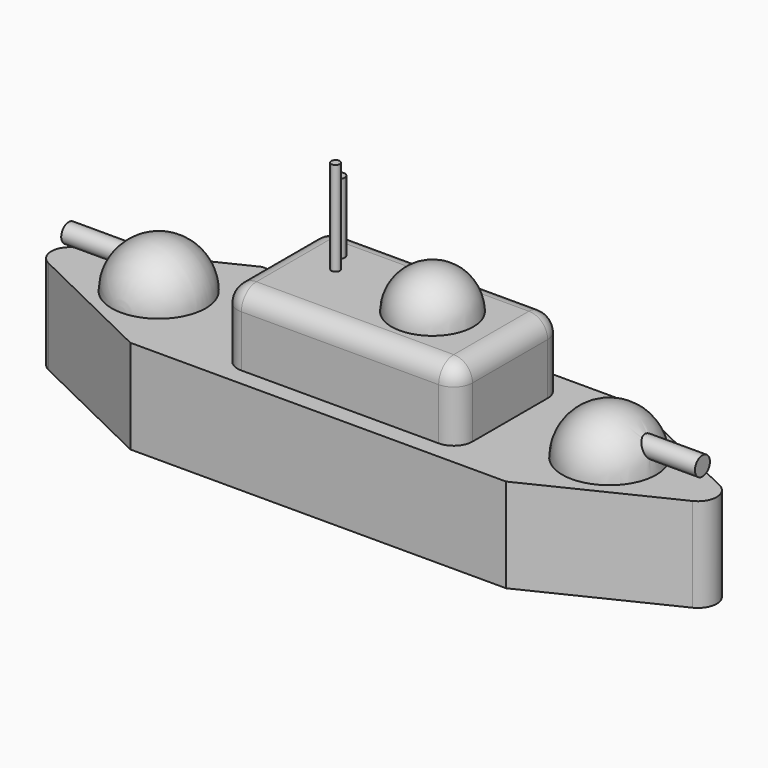
from build123d import *

# Parameters (mm, degrees)
F1_DEPTH  = 25.4
F2_W      = 63.5
F2_H      = 35.56
F3_DEPTH  = 19.05
F9_R      = 2.54
F10_DEPTH = 19.05
F12_R     = 2.54
F13_DEPTH = 19.05
F14_R     = 5.08
F15_R     = 5.08
F16_R     = 1.5271638032
F17_DEPTH = 19.05
F18_R     = 1.1438569205
F19_DEPTH = 25.4


# Not quite as in the source:
# - the program builds the solid bodies; features that only make, move or delete a surface that nothing else refers to are left out


with BuildPart() as f1:
    # F0 (on Top) → F1 (new body)
    with BuildSketch(Plane.XY):
        Polygon((-109.4730429574, -7.8658423934), (-63.7924405375, -30.0902110584), (37.8075594625, -30.0902110584), (83.4881618824, -7.8658423934), (37.8075594625, 14.3585262716), (-63.7924405375, 14.3585262716), align=None)
    extrude(amount=F1_DEPTH)

    # F2 (on face) → F3 (join)
    with BuildSketch(Plane.XY.offset(25.4)):
        with Locations((-10.9020974487, -7.5584737481)):
            Rectangle(F2_W, F2_H)
    extrude(amount=F3_DEPTH)

    # F5 (on face) → F6 (revolve)
    with BuildSketch(Plane.XY.offset(25.4)):
        with BuildLine():
            Line((-73.9079761496, 4.8341565959), (-73.9079761496, -20.5658413827))
            ThreePointArc((-73.9079761496, -20.5658413827), (-61.2130429574, -7.8658423934), (-73.9079761496, 4.8341565959))
        make_face()
    revolve(axis=Axis((-73.9079761496, -7.8658423934, 25.4), (0, 1, 0)))

    # F4 (on face) → F7 (revolve)
    with BuildSketch(Plane.XY.offset(25.4)):
        with BuildLine():
            Line((47.92816229, -7.8712259838), (47.92816229, 4.8287740162))
            ThreePointArc((47.92816229, 4.8287740162), (35.22816229, -7.8712259838), (47.92816229, -20.5712259838))
            Line((47.92816229, -20.5712259838), (47.92816229, -7.8712259838))
        make_face()
    revolve(axis=Axis((47.92816229, -7.8712259838, 25.4), (0, 1, 0)))

    # F9 (on offset) → F10 (join)
    with BuildSketch(Plane.YZ.offset(53.848)):
        with Locations((-7.6085058972, 31.3998050988)):
            Circle(F9_R)
    extrude(amount=F10_DEPTH)

    # F12 (on offset) → F13 (join)
    with BuildSketch(Plane.YZ.offset(-79.248)):
        with Locations((-7.7845989726, 31.3248895109)):
            Circle(F12_R)
    extrude(amount=-F13_DEPTH)

    # F14
    f14_edges = [f1.edges().sort_by_distance(p)[0] for p in [
        (-42.652097, -7.558474, 44.45),
        (-10.902097, -25.338474, 44.45),
        (-10.902097, 10.221526, 44.45),
        (20.847903, -7.558474, 44.45),
        (-42.652097, -25.338474, 34.925),
        (20.847903, -25.338474, 34.925),
        (20.847903, 10.221526, 34.925),
        (-42.652097, 10.221526, 34.925),
    ]]
    fillet(f14_edges, radius=F14_R)

    # F15
    f15_edges = [f1.edges().sort_by_distance(p)[0] for p in [
        (-109.473043, -7.865842, 12.7),
        (83.488162, -7.865842, 12.7),
    ]]
    fillet(f15_edges, radius=F15_R)

    # F16 (on face) → F17 (join)
    with BuildSketch(Plane.XY.offset(44.45)):
        with Locations((-31.4132720232, 0)):
            Circle(F16_R)
    extrude(amount=F17_DEPTH)

    # F18 (on face) → F19 (join)
    with BuildSketch(Plane.XY.offset(44.45)):
        with Locations((-28.1017310917, -5.3548677824)):
            Circle(F18_R)
    extrude(amount=F19_DEPTH)

    # F20 (on face) → F21 (revolve)
    with BuildSketch(Plane.XY.offset(44.45)):
        with BuildLine():
            Line((0, -7.7205132693), (0, -18.7808952404))
            ThreePointArc((0, -18.7808952404), (11.0603819711, -7.7205132693), (0, 3.3398687018))
            Line((0, 3.3398687018), (0, -7.7205132693))
        make_face()
    revolve(axis=Axis((0, -13.2507042548, 44.45), (0, 1, 0)))


solid = f1.part
